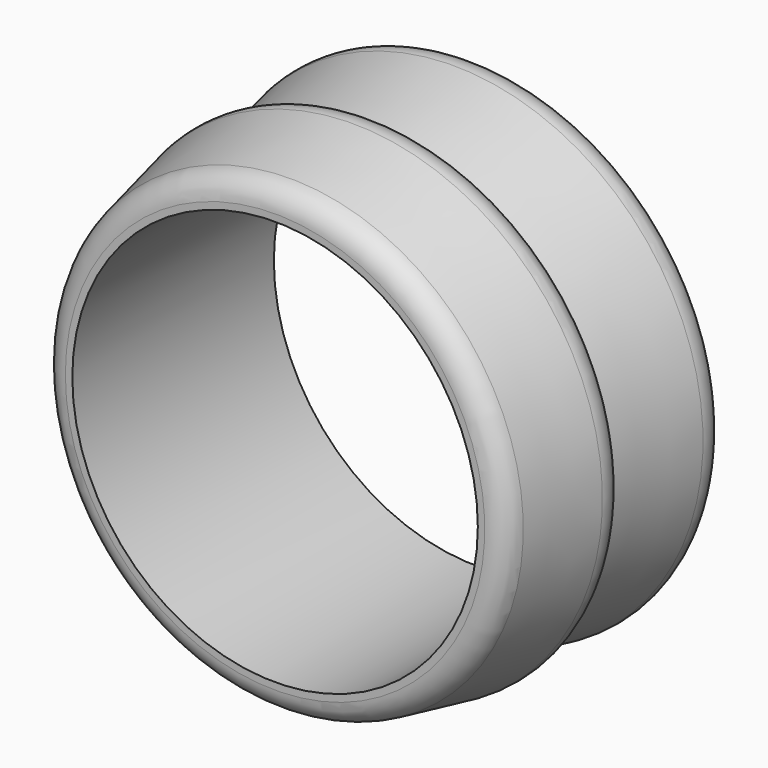
from build123d import *


# Not quite as in the source:
# - a fillet or chamfer that OpenCascade refuses, or shapes differently, is made with other operations: its cross-section is extruded or revolved along the edge and cut away or added


with BuildPart() as f1:
    # F0 (on Top) → F1 (revolve)
    with BuildSketch(Plane.XY):
        Polygon((11.0400244594, -26.4020487666), (11.0400244594, 26.4020487666), (5.5200122297, 26.4020487666), (5.5200122297, 0), (5.5200122297, -26.4020487666), align=None)
        Polygon((0, 0), (5.5200122297, -26.4020487666), (5.5200122297, 0), align=None)
        Polygon((5.5200122297, 0), (5.5200122297, 26.4020487666), (0, 26.4020487666), align=None)
    revolve(axis=Axis((53.5406768322, 0, 0), (0, -1, 0)))

    # F2: fillet of radius 5 on 3 edges, made by hand

    # F2_s1 → F2_t2 (revolve, cut)
    with BuildSketch(Plane.XY):
        with BuildLine():
            ThreePointArc((6.1534879532, 26.4020487666), (2.2730077773, 24.5551224424), (1.2593119965, 20.3787982085))
            Line((1.2593119965, 20.3787982085), (0, 26.4020487666))
            Line((0, 26.4020487666), (6.1534879532, 26.4020487666))
        make_face()
    revolve(axis=Axis((53.5406768322, 26.4020487666, 0), (0, -1, 0)), mode=Mode.SUBTRACT)

    # F2_s3 → F2_t4 (revolve, cut)
    with BuildSketch(Plane.XY):
        with BuildLine():
            ThreePointArc((5.5200122297, 0), (2.0748843765, -2.0569822638), (1.2511057448, -5.9840003086))
            Line((1.2511057448, -5.9840003086), (0, 0))
            Line((0, 0), (5.5200122297, 0))
        make_face()
    revolve(axis=Axis((53.5406768322, 0, 0), (0, -1, 0)), mode=Mode.SUBTRACT)

    # F2_s5 → F2_t6 (revolve, cut)
    with BuildSketch(Plane.XY):
        with BuildLine():
            ThreePointArc((4.6885727551, -22.4252993247), (6.4296750361, -25.2825289425), (9.5827487118, -26.4020487666))
            Line((9.5827487118, -26.4020487666), (5.5200122297, -26.4020487666))
            Line((5.5200122297, -26.4020487666), (4.6885727551, -22.4252993247))
        make_face()
    revolve(axis=Axis((53.5406768322, -26.4020487666, 0), (0, -1, 0)), mode=Mode.SUBTRACT)


solid = f1.part
